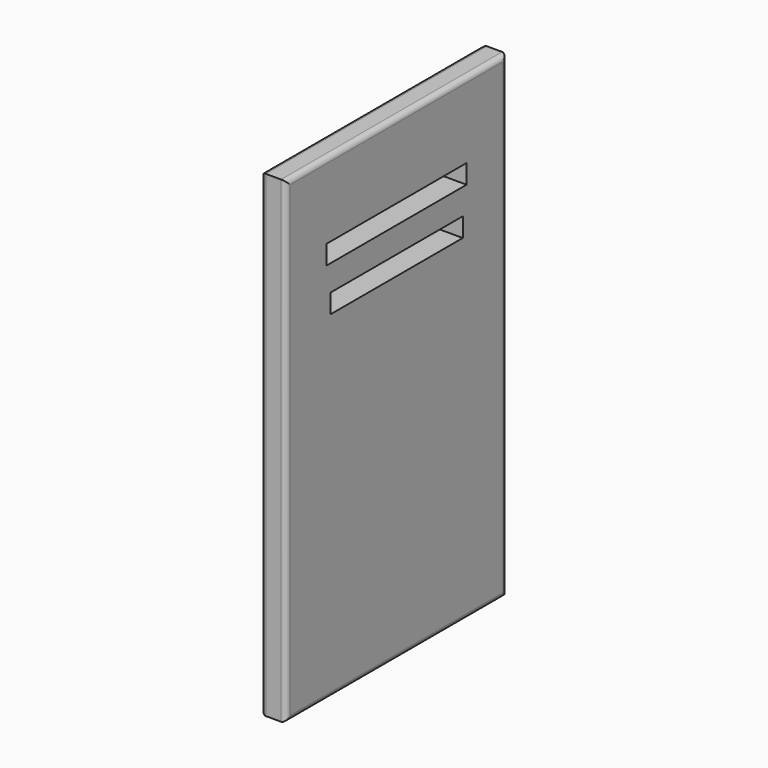
from build123d import *

# Parameters (mm, degrees)
F0_W         = 279.4
F0_H         = 482.6
F1_DEPTH     = 25.4
F2_R         = 5.08
F3_R         = 5.08
F4_W         = 176.9686788321
F4_H         = 19.3408131599
F5_DEPTH     = 25.4
F6_W         = 167.2982573509
F6_H         = 19.3408429623
F7_DEPTH     = 25.4
F8_W         = 152.4
F8_H         = 152.4
F9_DEPTH     = 25.4
F10_T        = 2.54
F10_T3_DEPTH = 157.48
F10_T5_DEPTH = 157.48
F10_T7_DEPTH = 30.48
F11_W        = 39.6487191319
F11_H        = 63.5
F12_DEPTH    = 25.4
F13_R        = 7.7119354401
F14_DEPTH    = 50.8


# Not quite as in the source:
# - a shell that OpenCascade refuses in one call is made with other operations: the cavity is built on its own and cut out


with BuildPart() as f1:
    # F0 (on Right) → F1 (new body)
    with BuildSketch(Plane.YZ):
        Rectangle(F0_W, F0_H)
    extrude(amount=F1_DEPTH)

    # F2
    f2_edges = [f1.edges().sort_by_distance(p)[0] for p in [
        (0, 139.7, 0),
        (0, 0, 241.3),
        (0, -139.7, 0),
        (0, 0, -241.3),
    ]]
    fillet(f2_edges, radius=F2_R)

    # F3
    f3_edges = [f1.edges().sort_by_distance(p)[0] for p in [
        (25.4, 139.7, 0),
        (25.4, 0, 241.3),
        (25.4, -139.7, 0),
        (25.4, 0, -241.3),
    ]]
    fillet(f3_edges, radius=F3_R)

    # F4 (on face) → F5 (cut)
    with BuildSketch(Plane(origin=(0, 0, 0), x_dir=(0, -1, 0), z_dir=(-1, 0, 0))):
        with Locations((0, 155.2102416754)):
            Rectangle(F4_W, F4_H)
    extrude(amount=-F5_DEPTH, mode=Mode.SUBTRACT)

    # F6 (on face) → F7 (cut)
    with BuildSketch(Plane.YZ.offset(25.4)):
        with Locations((0, 109.7592636943)):
            Rectangle(F6_W, F6_H)
    extrude(amount=-F7_DEPTH, mode=Mode.SUBTRACT)

    # F8 (on face) → F9 (join)
    with BuildSketch(Plane(origin=(0, 0, 0), x_dir=(0, -1, 0), z_dir=(-1, 0, 0))):
        Rectangle(F8_W, F8_H)
    extrude(amount=F9_DEPTH)

    # F10: shell of thickness 2.54, made by hand


with BuildPart() as f10_core1:
    # F10_t2: copy of F1
    add(f1.part)

    # the walls: a layer under each face that stays
    f10_faces = [f10_core1.faces().sort_by_distance(p)[0] for p in [
        (12.7, 139.7, 0),
        (12.7, 0, -241.3),
        (23.912103095, 138.2121018019, 0),
        (1.4878975516, 138.2121024484, 0),
        (12.7, 0, 241.3),
        (12.7, -139.7, 0),
        (23.912103095, 0, -239.8121018019),
        (1.4878975516, 0, -239.8121024484),
        (25.4, 0, 0),
        (23.912103095, 0, 239.8121018019),
        (0, -89.7466666667, -157.48),
        (1.4878975516, 0, 239.8121024484),
        (23.912103095, -138.2121018019, 0),
        (1.4878975516, -138.2121024484, 0),
        (12.7, 0, 119.4296851754),
        (12.7, -83.6491286755, 109.7592636943),
        (12.7, 0, 100.0888422132),
        (12.7, 83.6491286755, 109.7592636943),
        (12.7, -88.484339416, 155.2102416754),
        (12.7, 0, 145.5398350954),
        (12.7, 0, 164.8806482553),
        (12.7, 88.484339416, 155.2102416754),
        (-12.7, -76.2, 0),
        (-12.7, 0, -76.2),
        (-12.7, 76.2, 0),
        (-12.7, 0, 76.2),
    ]]
    thicken(f10_faces, amount=-F10_T, mode=Mode.SUBTRACT)

    # F10_s4 → F10_t3 (cut)
    with BuildSketch(Plane.XY.offset(-78.74)):
        Polygon((-0.0254, -76.2254), (2.54, -76.2), (2.54, -73.66), (0, -73.66), align=None)
        Polygon((-0.0254, 76.2254), (2.54, 76.2), (2.54, 73.66), (0, 73.66), align=None)
    extrude(amount=F10_T3_DEPTH, mode=Mode.SUBTRACT)

    # F10_s6 → F10_t5 (cut)
    with BuildSketch(Plane.XZ.offset(-78.74)):
        Polygon((-0.0254, -76.2254), (2.54, -76.2), (2.54, -73.66), (0, -73.66), align=None)
        Polygon((-0.0254, 76.2254), (2.54, 76.2), (2.54, 73.66), (0, 73.66), align=None)
    extrude(amount=F10_T5_DEPTH, mode=Mode.SUBTRACT)

    # F10_s8 → F10_t7 (cut)
    with BuildSketch(Plane.YZ.offset(-2.54)):
        Polygon((83.6237286755, 119.4042851754), (83.6491286755, 121.9696851754), (86.1891286755, 121.9696851754), (86.1891286755, 119.4296851754), align=None)
        Polygon((-83.6237286755, 119.4042851754), (-83.6491286755, 121.9696851754), (-86.1891286755, 121.9696851754), (-86.1891286755, 119.4296851754), align=None)
        Polygon((-83.6237286755, 100.1142422132), (-86.1891286755, 100.0888422132), (-86.1891286755, 97.5488422132), (-83.6491286755, 97.5488422132), align=None)
        Polygon((83.6237286755, 100.1142422132), (83.6491286755, 97.5488422132), (86.1891286755, 97.5488422132), (86.1891286755, 100.0888422132), align=None)
        Polygon((-88.458939416, 145.5652350954), (-91.024339416, 145.5398350954), (-91.024339416, 142.9998350954), (-88.484339416, 142.9998350954), align=None)
        Polygon((-88.458939416, 164.8552482553), (-91.024339416, 164.8806482553), (-91.024339416, 167.4206482553), (-88.484339416, 167.4206482553), align=None)
        Polygon((88.458939416, 145.5652350954), (88.484339416, 142.9998350954), (91.024339416, 142.9998350954), (91.024339416, 145.5398350954), align=None)
        Polygon((88.458939416, 164.8552482553), (88.484339416, 167.4206482553), (91.024339416, 167.4206482553), (91.024339416, 164.8806482553), align=None)
    extrude(amount=F10_T7_DEPTH, mode=Mode.SUBTRACT)


with BuildPart() as f1_1:
    add(f1.part)

    # what is left inside the walls is the cavity
    f10_cavity = [f10_core1.part.solids().sort_by_distance(p)[0] for p in [
        (22.8346, 0, -78.74),
    ]]
    add(f10_cavity, mode=Mode.SUBTRACT)

    # F11 (on face) → F12 (join)
    with BuildSketch(Plane(origin=(0, 0, 0), x_dir=(0, -1, 0), z_dir=(-1, 0, 0))):
        with Locations((0, 44.45)):
            Rectangle(F11_W, F11_H)
    extrude(amount=F12_DEPTH)

    # F13 (on face) → F14 (cut)
    with BuildSketch(Plane(origin=(0, 19.824359566, 0), x_dir=(-1, 0, 0), z_dir=(0, 1, 0))):
        with Locations((12.3025374487, 43.18)):
            Circle(F13_R)
    extrude(amount=-F14_DEPTH, mode=Mode.SUBTRACT)


solid = f1_1.part
